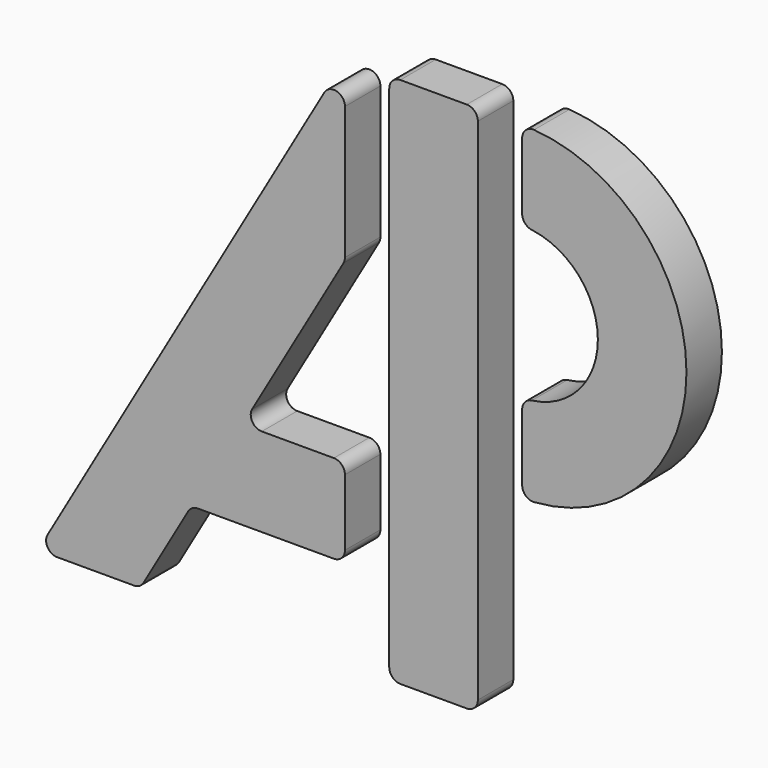
from build123d import *

# Parameters (mm, degrees)
F2_DEPTH = 6.35
F3_R     = 1.5875
F3_2_R   = 1.5875
F3_3_R   = 1.5875


# Not quite as in the source:
# - a variable given as a bare number and used for a length is read in inches; the dataset says mm whatever the document's units were


with BuildPart() as f2:
    # F1 (on Front) → F2 (new body)
    with BuildSketch(Plane.XZ):
        Polygon((-12.7, 12.7), (-12.7, 38.1), (-56.6940905122, -38.1), (-42.0293936748, -38.1), (-34.6970452561, -25.4), (-27.3646968374, -12.7), align=None)
        Polygon((-12.7, -25.4), (-12.7, -12.7), (-27.3646968374, -12.7), (-34.6970452561, -25.4), align=None)
    extrude(amount=F2_DEPTH)

    # F3
    f3_edges = [f2.edges().sort_by_distance(p)[0] for p in [
        (-12.7, -3.175, 38.1),
        (-12.7, -3.175, 12.7),
        (-12.7, -3.175, -25.4),
        (-34.697045, -3.175, -25.4),
        (-42.029394, -3.175, -38.1),
        (-56.694091, -3.175, -38.1),
        (-27.364697, -3.175, -12.7),
        (-12.7, -3.175, -12.7),
    ]]
    fillet(f3_edges, radius=F3_R)


with BuildPart() as f2b:
    # F1 (on Front) → F2, piece 2 (new body)
    with BuildSketch(Plane.XZ):
        Polygon((6.35, 38.1), (-6.35, 38.1), (-6.35, 12.7), (-6.35, -12.7), (-6.35, -25.4), (-6.35, -38.1), (6.35, -38.1), (6.35, -8.9941899428), (6.35, 3.7058100572), (6.35, 25.4), align=None)
    extrude(amount=F2_DEPTH)

    # F3#2
    f3_2_edges = [f2b.edges().sort_by_distance(p)[0] for p in [
        (-6.35, -3.175, 38.1),
        (6.35, -3.175, 38.1),
        (-6.35, -3.175, -38.1),
        (6.35, -3.175, -38.1),
    ]]
    fillet(f3_2_edges, radius=F3_2_R)


with BuildPart() as f2c:
    # F1 (on Front) → F2, piece 3 (new body)
    with BuildSketch(Plane.XZ):
        with BuildLine():
            ThreePointArc((12.7, -8.9941899428), (36.2470949714, 14.5529050286), (12.7, 38.1))
            Line((12.7, 38.1), (12.7, 25.4))
            ThreePointArc((12.7, 25.4), (23.5470949714, 14.5529050286), (12.7, 3.7058100572))
            Line((12.7, 3.7058100573), (12.7, -8.9941899428))
        make_face()
    extrude(amount=F2_DEPTH)

    # F3#3
    f3_3_edges = [f2c.edges().sort_by_distance(p)[0] for p in [
        (12.7, -3.175, -8.99419),
        (12.7, -3.175, 3.70581),
        (12.7, -3.175, 25.4),
        (12.7, -3.175, 38.1),
    ]]
    fillet(f3_3_edges, radius=F3_3_R)


solid = Compound([f2.part, f2b.part, f2c.part])
